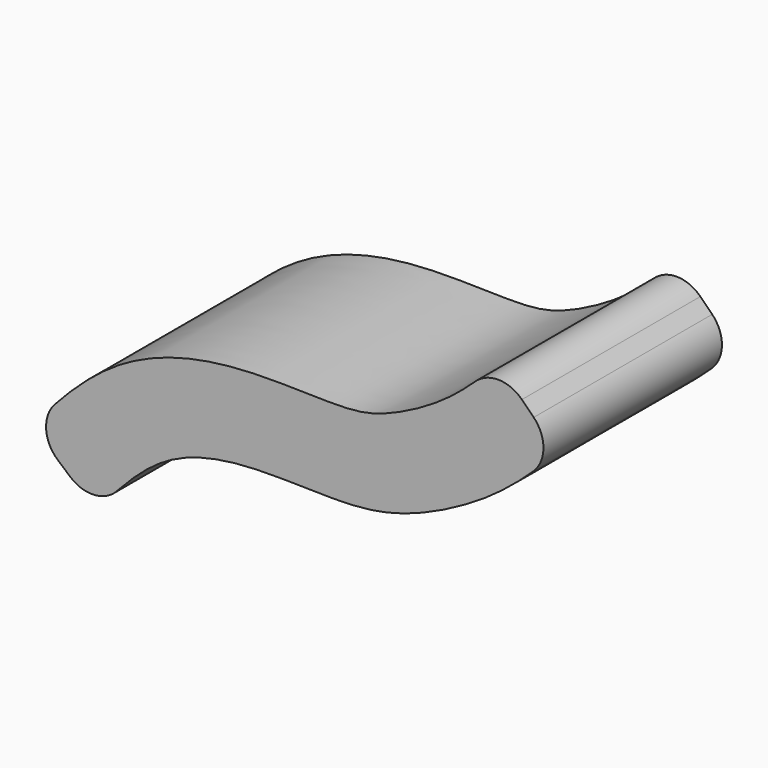
from build123d import *

# Parameters (mm, degrees)
F1_DEPTH = 50.8
F2_R     = 7.62


# Not quite as in the source:
# - the dataset's text gives a spline's control points without its knots; the knots are read off the source's solid


with BuildPart() as f1:
    # F0 (on Front) → F1 (new body)
    with BuildSketch(Plane.XZ):
        with BuildLine():
            Line((-51.4566205376, -7.6382097449), (-37.0489656925, -20.1010350138))
            add(Edge.make_bspline(
                [(-37.0489656925, -20.1010350138), (-32.0961571271, -14.3753384093), (-22.4411994409, -3.2137201658), (-2.567876156, 1.0362784201), (19.8507775599, -0.7305766437), (35.0126136642, 1.7996710925), (54.6374865112, 12.120662721), (63.7504331122, 21.1999324541), (68.1858584285, 25.6189666688)],
                knots=[0, 0, 0, 0, 0.1744362409, 0.340044341, 0.5157839146, 0.662689084, 0.8358250694, 1, 1, 1, 1], degree=3))
            Line((68.1858584285, 25.6189666688), (54.7404326534, 39.1142642774))
            add(Edge.make_bspline(
                [(-51.4566205376, -7.6382097449), (-50.569332054, -6.6124594882), (-48.7206333421, -4.4744710724), (-45.6807379161, -1.083016907), (-42.8655113291, 1.8341952687), (-40.3934284717, 4.1792576456), (-38.413862066, 5.9302516977), (-36.2924687687, 7.6576678013), (-34.392168296, 9.0614262042), (-32.7845564877, 10.1507045755), (-31.5329658928, 10.9476488916), (-30.2357008088, 11.7189891488), (-28.9317170147, 12.440929508), (-27.6164352854, 13.1185008592), (-25.8531615823, 13.961984086), (-22.7482671671, 15.2847678022), (-18.2999008711, 16.7576548912), (-13.9122537643, 17.7575537331), (-10.4620230508, 18.3293395163), (-7.9060318762, 18.6573853028), (-5.3849265205, 18.8972362958), (-2.8912531141, 19.060728488), (-0.4571417194, 19.1579367871), (2.6992657096, 19.2188727368), (6.4751057026, 19.1986064325), (10.688599572, 19.1069677477), (13.872523357, 19.034713831), (16.1671624828, 19.0086227881), (17.4801550196, 19.0099656248), (18.4476603272, 19.0234519818), (19.126692671, 19.0398701949), (19.7635064415, 19.0627895847), (20.5708993056, 19.1021374284), (21.5017087851, 19.1671291568), (22.853887137, 19.3033614178), (24.3475932959, 19.5320424193), (25.7829635166, 19.8577835208), (27.0218215144, 20.2115138008), (28.0214471049, 20.5347589257), (29.1187561712, 20.9292509093), (30.7086380041, 21.5547332667), (32.8673205533, 22.5055753198), (35.5872650511, 23.8682182699), (37.8559849368, 25.1420412869), (39.6138298192, 26.2132708199), (40.8886976676, 27.0336077895), (42.1078319952, 27.8629622939), (43.2480720812, 28.68464647), (44.37217855, 29.5417355035), (45.8540278008, 30.7312919433), (47.6956238749, 32.3155185334), (50.6875135665, 35.0808060073), (53.0519039531, 37.4319755301), (54.7404326534, 39.1142642774)],
                knots=[0, 0, 0, 0, 0.03125, 0.0625, 0.09375, 0.109375, 0.125, 0.140625, 0.15625, 0.1640625, 0.171875, 0.1796875, 0.1875, 0.1953125, 0.203125, 0.21875, 0.25, 0.28125, 0.296875, 0.3125, 0.328125, 0.34375, 0.359375, 0.375, 0.40625, 0.4375, 0.46875, 0.484375, 0.5, 0.5078125, 0.515625, 0.5234375, 0.53125, 0.546875, 0.5625, 0.59375, 0.625, 0.640625, 0.65625, 0.671875, 0.6875, 0.71875, 0.75, 0.78125, 0.796875, 0.8125, 0.828125, 0.84375, 0.859375, 0.875, 0.90625, 0.9375, 1, 1, 1, 1], degree=3))
        make_face()
    extrude(amount=F1_DEPTH)

    # F2
    f2_edges = [f1.edges().sort_by_distance(p)[0] for p in [
        (54.740433, -25.4, 39.114264),
        (68.185858, -25.4, 25.618967),
        (-51.456621, -25.4, -7.63821),
        (-37.048966, -25.4, -20.101035),
    ]]
    fillet(f2_edges, radius=F2_R)


solid = f1.part
